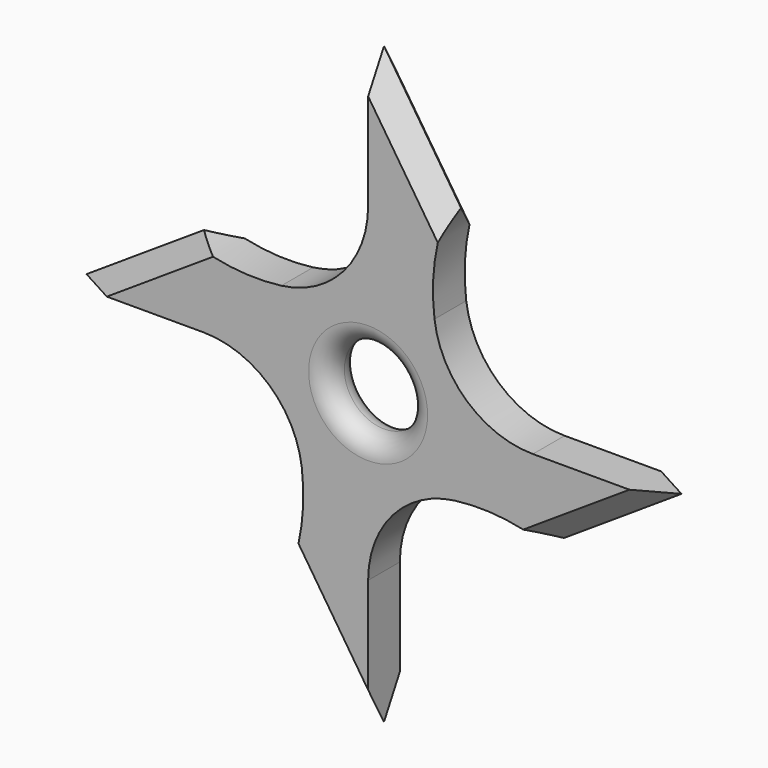
from build123d import *

# Parameters (mm, degrees)
F1_DEPTH = 5.08
F2_R     = 5.08
F3_DEPTH = 25.4
F4_R     = 12.7
F5_SIZE  = 2.53999
F6_R     = 2.53999


# Not quite as in the source:
# - a fillet or chamfer is up to 0.001 mm smaller than in the source, because OpenCascade refuses the exact size


with BuildPart() as f1:
    # F0 (on Front) → F1 (new body)
    with BuildSketch(Plane.XZ):
        with BuildLine():
            Line((-12.7, 0), (0, 0))
            Line((0, 0), (0, 12.7))
            ThreePointArc((0, 12.7), (-11.1850810666, 8.4922018267), (-23.0563643922, 9.8648766371))
            Line((-23.0563643922, 9.8648766371), (-38.1, 0))
            Line((-38.1, 0), (-12.7, 0))
        make_face()
        with BuildLine():
            Line((0, 12.7), (0, 0))
            Line((0, 0), (12.7, 0))
            ThreePointArc((12.7, 0), (8.4922018267, 11.1850810666), (9.8648766371, 23.0563643922))
            Line((9.8648766371, 23.0563643922), (0, 38.1))
            Line((0, 38.1), (0, 12.7))
        make_face()
        with BuildLine():
            Line((0, -12.7), (0, 0))
            Line((0, 0), (-12.7, 0))
            ThreePointArc((-12.7, 0), (-8.4922018267, -11.1850810666), (-9.8648766371, -23.0563643922))
            Line((-9.8648766371, -23.0563643922), (0, -38.1))
            Line((0, -38.1), (0, -12.7))
        make_face()
        with BuildLine():
            Line((12.7, 0), (0, 0))
            Line((0, 0), (0, -12.7))
            ThreePointArc((0, -12.7), (11.1850810666, -8.4922018267), (23.0563643922, -9.8648766371))
            Line((23.0563643922, -9.8648766371), (38.1, 0))
            Line((38.1, 0), (12.7, 0))
        make_face()
    extrude(amount=F1_DEPTH)

    # F2 (on face) → F3 (cut)
    with BuildSketch(Plane.XZ.offset(5.08)):
        Circle(F2_R)
    extrude(amount=-F3_DEPTH, mode=Mode.SUBTRACT)

    # F4
    f4_edges = [f1.edges().sort_by_distance(p)[0] for p in [
        (0, -2.54, 12.7),
        (12.7, -2.54, 0),
        (0, -2.54, -12.7),
        (-12.7, -2.54, 0),
    ]]
    fillet(f4_edges, radius=F4_R)

    # F5 (size 2.54 in the source; OpenCascade refuses exactly that, so slightly less here)
    f5_edges = [f1.edges().sort_by_distance(p)[0] for p in [
        (30.578182, 0, -4.932438),
        (30.578182, -5.08, -4.932438),
        (4.932438, 0, 30.578182),
        (4.932438, -5.08, 30.578182),
        (-4.932438, 0, -30.578182),
        (-4.932438, -5.08, -30.578182),
        (-30.578182, 0, 4.932438),
        (-30.578182, -5.08, 4.932438),
    ]]
    chamfer(f5_edges, length=F5_SIZE)

    # F6 (radius 2.54 in the source; OpenCascade refuses exactly that, so slightly less here)
    f6_edges = [f1.edges().sort_by_distance(p)[0] for p in [
        (-5.08, 0, 0),
        (-5.08, -5.08, 0),
    ]]
    fillet(f6_edges, radius=F6_R)


solid = f1.part
